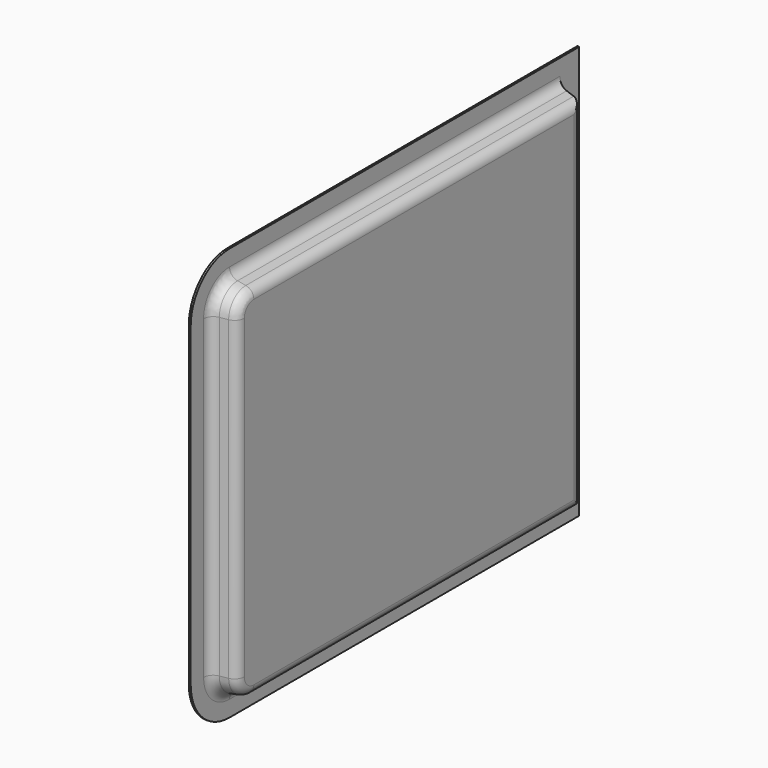
from build123d import *

# Parameters (mm, degrees)
F1_DEPTH               = 25
DRAFT_F1_DRAFTED_ANGLE = 10
F2_DEPTH               = 2
F3_R                   = 10


# Not quite as in the source:
# - an extrude with a draft is written as a straight extrude whose walls are then drafted


with BuildPart() as f1:
    # F0 (on Right) → F1 (new body)
    with BuildSketch(Plane.YZ):
        with BuildLine():
            Line((-200, -187.5), (225, -187.5))
            Line((225, -187.5), (225, 187.5))
            Line((225, 187.5), (-200, 187.5))
            ThreePointArc((-200, 187.5), (-217.6776695297, 180.1776695297), (-225, 162.5))
            Line((-225, 162.5), (-225, -162.5))
            ThreePointArc((-225, -162.5), (-217.6776695297, -180.1776695297), (-200, -187.5))
        make_face()
    extrude(amount=F1_DEPTH)

    # draft_F1_drafted
    draft_f1_drafted_walls = [f1.faces().sort_by_distance(p)[0] for p in [
        (16.6666666667, 12.5, -187.5),
        (16.6666666667, 225, 0),
        (16.6666666667, 12.5, 187.5),
        (16.6666666667, -217.6776695297, 180.1776695297),
        (16.6666666667, -225, 0),
        (16.6666666667, -217.6776695297, -180.1776695297),
    ]]
    draft(draft_f1_drafted_walls, neutral_plane=Plane.YZ, angle=DRAFT_F1_DRAFTED_ANGLE)

    # F0 (on Right) → F2 (join)
    with BuildSketch(Plane.YZ):
        with BuildLine():
            Line((-200, -212.5), (250, -212.5))
            Line((250, -212.5), (250, 212.5))
            Line((250, 212.5), (-200, 212.5))
            ThreePointArc((-200, 212.5), (-235.3553390593, 197.8553390593), (-250, 162.5))
            Line((-250, 162.5), (-250, -162.5))
            ThreePointArc((-250, -162.5), (-235.3553390593, -197.8553390593), (-200, -212.5))
        make_face()
        with BuildLine():
            Line((225, 187.5), (225, -187.5))
            Line((225, -187.5), (-200, -187.5))
            ThreePointArc((-200, -187.5), (-217.6776695297, -180.1776695297), (-225, -162.5))
            Line((-225, -162.5), (-225, 162.5))
            ThreePointArc((-225, 162.5), (-217.6776695297, 180.1776695297), (-200, 187.5))
            Line((-200, 187.5), (225, 187.5))
        make_face(mode=Mode.SUBTRACT)
        with BuildLine():
            Line((-200, -187.5), (225, -187.5))
            Line((225, -187.5), (225, 187.5))
            Line((225, 187.5), (-200, 187.5))
            ThreePointArc((-200, 187.5), (-217.6776695297, 180.1776695297), (-225, 162.5))
            Line((-225, 162.5), (-225, -162.5))
            ThreePointArc((-225, -162.5), (-217.6776695297, -180.1776695297), (-200, -187.5))
        make_face()
    extrude(amount=-F2_DEPTH)

    # F3
    f3_edges = [f1.edges().sort_by_distance(p)[0] for p in [
        (0, 12.5, -187.5),
        (0, 12.5, 187.5),
        (0, -217.67767, 180.17767),
        (0, -225, 0),
        (0, -217.67767, -180.17767),
        (25, 10.295913, -183.091825),
        (25, 220.591825, 0),
        (25, 10.295913, 183.091825),
        (25, -214.560619, 177.060619),
        (25, -220.591825, 0),
        (25, -214.560619, -177.060619),
    ]]
    fillet(f3_edges, radius=F3_R)


solid = f1.part
